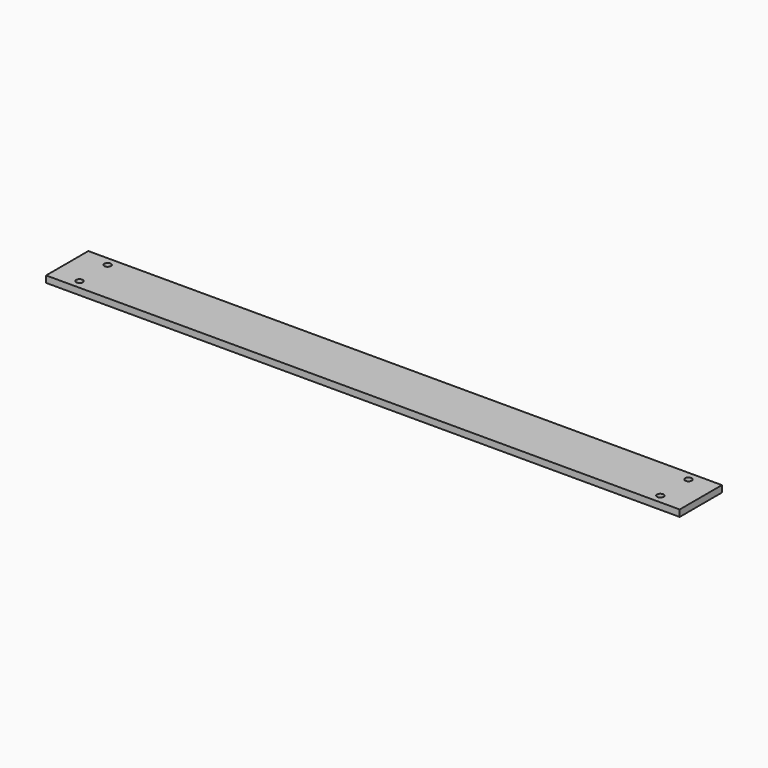
from build123d import *

# Parameters (mm, degrees)
F0_W     = 457.2
F0_H     = 38.1
F0_R     = 2.38125
F1_DEPTH = 4.7625


# Not quite as in the source:
# - a length typed as a fraction of an inch, garbled in the dataset ("3 / 203.2 mm" for 3/8 in), is restored


with BuildPart() as f1:
    # F0 (on Top) → F1 (new body)
    with BuildSketch(Plane.XY):
        Rectangle(F0_W, F0_H)
        with Locations((-209.55, -12.7)):
            Circle(F0_R, mode=Mode.SUBTRACT)
        with Locations((209.55, -12.7)):
            Circle(F0_R, mode=Mode.SUBTRACT)
        with Locations((-209.55, 12.7)):
            Circle(F0_R, mode=Mode.SUBTRACT)
        with Locations((209.55, 12.7)):
            Circle(F0_R, mode=Mode.SUBTRACT)
    extrude(amount=F1_DEPTH)


solid = f1.part
